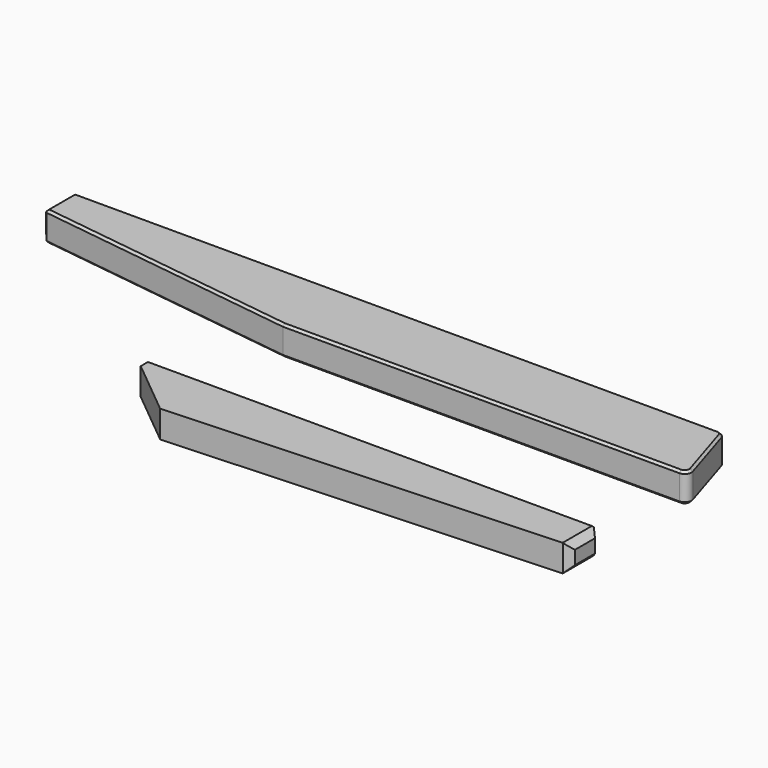
from build123d import *

# Parameters (mm, degrees)
F1_DEPTH    = 13
F2_R        = 3
F3_T1_DEPTH = 31.4300979278
F3_T3_DEPTH = 28.4300979278
F3_T5_DEPTH = 26.5899249285
F4_SIZE     = 1
F6_DEPTH    = 12
F7_SIZE     = 1
F8_T1_DEPTH = 31.4300979278
F8_T3_DEPTH = 25.4300979278
F8_T5_DEPTH = 26.709280871


# Not quite as in the source:
# - a fillet or chamfer that OpenCascade refuses, or shapes differently, is made with other operations: its cross-section is extruded or revolved along the edge and cut away or added


with BuildPart() as f1:
    # F0 (on Top) → F1 (new body)
    with BuildSketch(Plane.XY):
        Polygon((-180, 0), (0, 0), (-10, 32), (-300, 32), (-300, 16), align=None)
    extrude(amount=F1_DEPTH)

    # F2
    f2_edges = [f1.edges().sort_by_distance(p)[0] for p in [
        (-10, 32, 6.5),
        (0, 0, 6.5),
    ]]
    fillet(f2_edges, radius=F2_R)

    # F3: chamfer of 3 on 4 edges, made by hand

    # F3_s2 → F3_t1 (cut)
    with BuildSketch(Plane.XZ.offset(-39.7150489639)):
        Polygon((-297, 13), (-300, 10), (-300, 13), align=None)
        Polygon((-297, 0), (-300, 3), (-300, 0), align=None)
    extrude(amount=F3_T1_DEPTH, mode=Mode.SUBTRACT)

    # F3_s4 → F3_t3 (cut)
    with BuildSketch(Plane.XY.offset(-7.7150489639)):
        Polygon((-300, 29), (-297, 32), (-300, 32), align=None)
    extrude(amount=F3_T3_DEPTH, mode=Mode.SUBTRACT)

    # F3_s6 → F3_t5 (cut)
    with BuildSketch(Plane.XY.offset(-6.7949624643)):
        Polygon((-297.3964911603, 15.652865488), (-300, 18.6265491901), (-300, 16), align=None)
    extrude(amount=F3_T5_DEPTH, mode=Mode.SUBTRACT)

    # F4
    f4_edges = [f1.edges().sort_by_distance(p)[0] for p in [
        (-154.602786, 32, 13),
        (-154.602786, 32, 0),
        (-238.5, 7.8, 13),
        (-92.040286, 0, 13),
        (-238.5, 7.8, 0),
        (-92.040286, 0, 0),
    ]]
    chamfer(f4_edges, length=F4_SIZE)


with BuildPart() as f6:
    # F5 (on Top) → F6 (new body)
    with BuildSketch(Plane.XY):
        Polygon((-174.7816593036, -74.6039791434), (0, -65.8648961782), (0, -48.8648961782), (-200, -48.8648961782), (-200, -53.8648961782), align=None)
    extrude(amount=F6_DEPTH)

    # F7
    f7_edges = [f6.edges().sort_by_distance(p)[0] for p in [
        (-100, -48.864896, 12),
        (-100, -48.864896, 0),
    ]]
    chamfer(f7_edges, length=F7_SIZE)

    # F8: chamfer of 3 on 4 edges, made by hand

    # F8_s2 → F8_t1 (cut)
    with BuildSketch(Plane.XZ.offset(42.1498472143)):
        Polygon((0, 9), (-3, 12), (0, 12), align=None)
        Polygon((0, 3), (-3, 0), (0, 0), align=None)
    extrude(amount=F8_T1_DEPTH, mode=Mode.SUBTRACT)

    # F8_s4 → F8_t3 (cut)
    with BuildSketch(Plane.XY.offset(-6.7150489639)):
        Polygon((0, -51.8648961782), (-3, -48.8648961782), (0, -48.8648961782), align=None)
    extrude(amount=F8_T3_DEPTH, mode=Mode.SUBTRACT)

    # F8_s6 → F8_t5 (cut)
    with BuildSketch(Plane.XY.offset(-7.3546404355)):
        Polygon((0, -63.0111485191), (-2.8501871492, -66.0074055357), (0, -65.8648961782), align=None)
    extrude(amount=F8_T5_DEPTH, mode=Mode.SUBTRACT)


solid = Compound([f1.part, f6.part])
